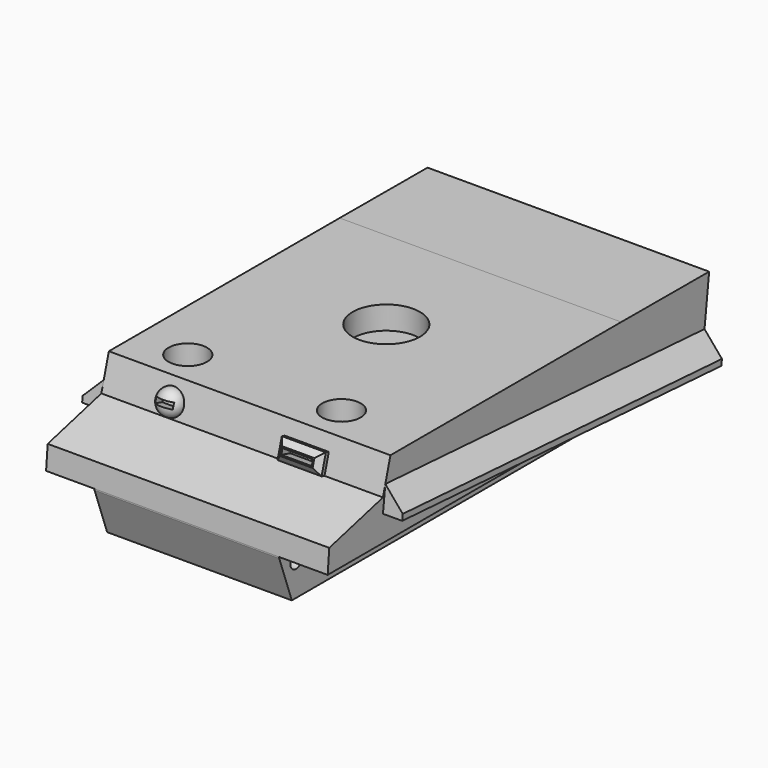
from build123d import *

# Parameters (mm, degrees)
F1_DEPTH      = 1859.28
F1_DEPTH_BACK = 1859.28
F3_DEPTH      = 1219.2
F3_DEPTH_BACK = 1219.2
F4_R          = 169.0151007429
F5_DEPTH      = 152.4
F6_R          = 152.39999
F7_W          = 227.70601511
F7_H          = 76.5184164047
F8_DEPTH      = 609.6
F9_W          = 581.4113616943
F9_H          = 259.9127333882
F10_DEPTH     = 127
F11_SIZE      = 76.2
F12_W         = 402.7016162872
F12_H         = 72.2321271896
F13_DEPTH     = 152.4
F14_R         = 254
F15_DEPTH     = 304.8
F16_R         = 444.5
F17_DEPTH     = 304.8
F19_DEPTH     = 254
F20_SIZE      = 253.99999
F22_DEPTH     = 254
F23_SIZE      = 253.99999
F24_R         = 95.25
F25_DEPTH     = 3048


# Not quite as in the source:
# - a fillet or chamfer is up to 0.001 mm smaller than in the source, because OpenCascade refuses the exact size


with BuildPart() as f1:
    # F0 (on Right) → F1 (new body, two sides)
    with BuildSketch(Plane.YZ) as f1_sk:
        Polygon((26.5650703895, 303.6401439784), (0, 0), (6181.2677383423, 0), (6297.168, 965.9386277199), (4846.1590473673, 969.9305323602), (1036.1590473673, 969.9305323602), (912.5677404125, 529.7521266595), align=None)
    extrude(amount=F1_DEPTH)
    extrude(f1_sk.sketch, amount=-F1_DEPTH_BACK)

    # F2 (on Right) → F3 (join, two sides)
    with BuildSketch(Plane.YZ) as f3_sk:
        Polygon((0, 0), (0, -16.3612399525), (208.4954793713, -589.1978615836), (6102.9406406674, -589.1978615836), (6181.4131736755, 0), align=None)
    extrude(amount=F3_DEPTH)
    extrude(f3_sk.sketch, amount=-F3_DEPTH_BACK)

    # F4 (on face) → F5 (join)
    with BuildSketch(Plane(origin=(0, 708.0104155563, -198.7919703987), x_dir=(1, 0, 0), z_dir=(0, -0.9627699162, 0.2703221937))):
        with Locations((-976.1219620705, 934.6183538437)):
            Circle(F4_R)
    extrude(amount=F5_DEPTH)

    # F6 (radius 152.4 in the source; OpenCascade refuses exactly that, so slightly less here)
    f6_edges = [f1.edges().sort_by_distance(p)[0] for p in [
        (-1145.137063, 813.932364, 742.227566),
    ]]
    fillet(f6_edges, radius=F6_R)

    # F7 (on face) → F8 (cut)
    with BuildSketch(Plane(origin=(0, 708.0104155563, -198.7919703987), x_dir=(1, 0, 0), z_dir=(0, -0.9627699162, 0.2703221937))):
        with Locations((-972.7734029293, 934.6184134483)):
            Rectangle(F7_W, F7_H)
    extrude(amount=F8_DEPTH, mode=Mode.SUBTRACT)

    # F9 (on face) → F10 (join)
    with BuildSketch(Plane(origin=(0, 708.0104155563, -198.7919703987), x_dir=(1, 0, 0), z_dir=(0, -0.9627699162, 0.2703221937))):
        with Locations((797.3860502243, 886.6730907796)):
            Rectangle(F9_W, F9_H)
    extrude(amount=F10_DEPTH)

    # F11
    f11_edges = [f1.edges().sort_by_distance(p)[0] for p in [
        (797.38605, 860.556141, 814.319206),
        (1088.091731, 825.426051, 689.201126),
        (797.38605, 790.295961, 564.083045),
        (506.680369, 825.426051, 689.201126),
    ]]
    chamfer(f11_edges, length=F11_SIZE)

    # F12 (on face) → F13 (cut)
    with BuildSketch(Plane(origin=(0, 585.738636195, -164.4610518002), x_dir=(1, 0, 0), z_dir=(0, -0.9627699162, 0.2703221937))):
        with Locations((796.0233688354, 885.5090737343)):
            Rectangle(F12_W, F12_H)
    extrude(amount=-F13_DEPTH, mode=Mode.SUBTRACT)

    # F14 (on face) → F15 (cut)
    with BuildSketch(Plane.XY.offset(969.9305323602)):
        with Locations((-1174.7832298279, 1483.3003282547)):
            Circle(F14_R)
        with Locations((839.1343951225, 1502.8530359268)):
            Circle(F14_R)
    extrude(amount=-F15_DEPTH, mode=Mode.SUBTRACT)

    # F16 (on face) → F17 (cut)
    with BuildSketch(Plane.XY.offset(969.9305323602)):
        with Locations((0, 3292.1198442413)):
            Circle(F16_R)
    extrude(amount=-F17_DEPTH, mode=Mode.SUBTRACT)

    # F18 (on face) → F19 (join)
    with BuildSketch(Plane.YZ.offset(1859.28)):
        Polygon((6220.8618148868, 329.9858638469), (951.8563702908, 669.6811142889), (912.5677404126, 339.6755581523), (6181.2677383423, 0), align=None)
    extrude(amount=F19_DEPTH)

    # F20 (size 254 in the source; OpenCascade refuses exactly that, so slightly less here)
    f20_edges = [f1.edges().sort_by_distance(p)[0] for p in [
        (2113.28, 3586.359093, 499.833489),
    ]]
    chamfer(f20_edges, length=F20_SIZE)

    # F21 (on face) → F22 (join)
    with BuildSketch(Plane(origin=(-1859.28, 0, 0), x_dir=(0, -1, 0), z_dir=(-1, 0, 0))):
        Polygon((-6220.8613622852, 329.9820917646), (-6181.2677383423, 0), (-912.5677404125, 339.7662410411), (-951.8803321296, 669.7664559221), align=None)
    extrude(amount=F22_DEPTH)

    # F23 (size 254 in the source; OpenCascade refuses exactly that, so slightly less here)
    f23_edges = [f1.edges().sort_by_distance(p)[0] for p in [
        (-2113.28, 3586.370847, 499.874274),
    ]]
    chamfer(f23_edges, length=F23_SIZE)

    # F24 (on face) → F25 (cut)
    with BuildSketch(Plane.YZ.offset(1219.2)):
        with Locations((278.1341671944, -156.8619608879)):
            Circle(F24_R)
        with Locations((834.8472714424, -386.4343762398)):
            Circle(F24_R)
        with Locations((1375.8672714424, -386.4343762398)):
            Circle(F24_R)
        with Locations((1916.8872714424, -386.4343762398)):
            Circle(F24_R)
        with Locations((2457.9072714424, -386.4343762398)):
            Circle(F24_R)
        with Locations((2998.9272714424, -386.4343762398)):
            Circle(F24_R)
        with Locations((3539.9472714424, -386.4343762398)):
            Circle(F24_R)
        with Locations((4080.9672714424, -386.4343762398)):
            Circle(F24_R)
        with Locations((4621.9872714424, -386.4343762398)):
            Circle(F24_R)
        with Locations((5163.0072714424, -386.4343762398)):
            Circle(F24_R)
        with Locations((5690.3038024902, -374.9557435513)):
            Circle(F24_R)
    extrude(amount=-F25_DEPTH, mode=Mode.SUBTRACT)


solid = f1.part
